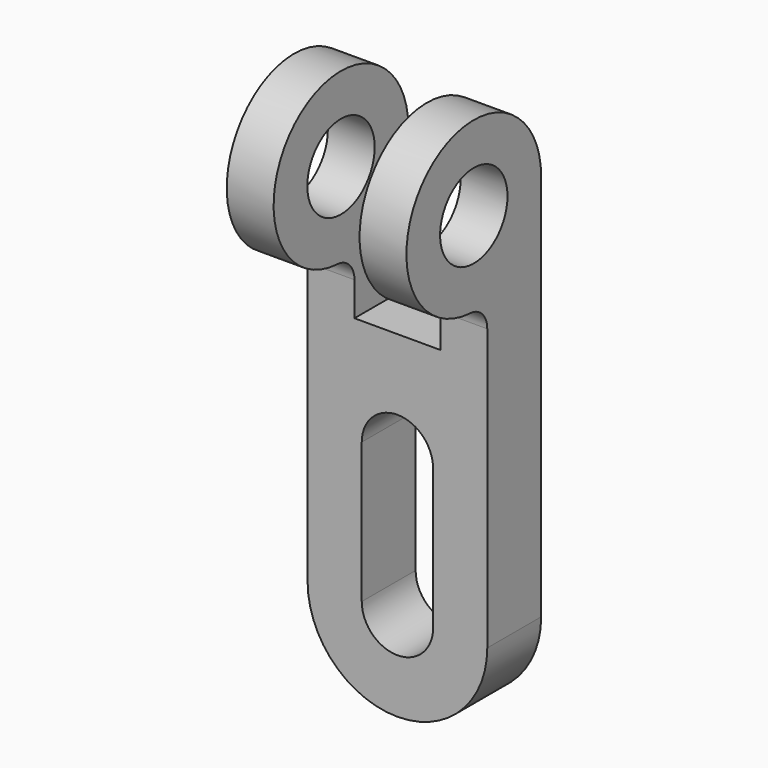
from build123d import *

# Parameters (mm, degrees)
F0_R     = 7.5
F1_DEPTH = 16
F3_W     = 15.3093371987
F3_H     = 50
F4_DEPTH = 55.501
F5_R     = 4
F6_DEPTH = 55.501


# Not quite as in the source:
# - a feature names something its author has since deleted; it is built from what else it names


with BuildPart() as f1:
    # F0 (on Right) → F1 (new body, symmetric)
    with BuildSketch(Plane.YZ):
        with BuildLine():
            Line((15, -85), (15, 0))
            ThreePointArc((15, 0), (-11.6189500386, 9.4868329805), (3, -14.6969384567))
            Line((3, -14.6969384567), (3, -85))
            Line((3, -85), (15, -85))
        make_face()
        Circle(F0_R, mode=Mode.SUBTRACT)
    extrude(amount=F1_DEPTH, both=True)

    # F3 (on offset) → F4 (cut, through all)
    with BuildSketch(Plane.XZ.offset(40.5)):
        with BuildLine():
            Line((6.3565325715, -68.9971852547), (6.3456283358, -44.3721764072))
            Line((6.3456283358, -44.3721764072), (6.3452962394, -43.6222039062))
            ThreePointArc((6.3452962394, -43.6222039062), (-0.1889815849, -37.6462766652), (-6.3565331947, -44))
            Line((-6.3565331947, -44), (-6.3565331947, -69))
            ThreePointArc((-6.3565331947, -69), (0, -75.3565331947), (6.3565331947, -69))
            ThreePointArc((6.3565331947, -69), (6.3565330389, -68.9985926273), (6.3565325715, -68.9971852547))
        make_face()
        Rectangle(F3_W, F3_H)
    extrude(amount=-F4_DEPTH, mode=Mode.SUBTRACT)

    # F5
    f5_edges = [f1.edges().sort_by_distance(p)[0] for p in [
        (-11.827334, 3, -14.696938),
        (11.827334, 3, -14.696938),
    ]]
    fillet(f5_edges, radius=F5_R)

    # F3 (on offset) → F6 (cut, through all)
    with BuildSketch(Plane.XZ.offset(40.5)):
        with BuildLine():
            ThreePointArc((2.313e-07, -85), (-11.3137084172, -80.3137085808), (-16, -69))
            Line((-16, -69), (-16, -85))
            Line((-16, -85), (2.313e-07, -85))
        make_face()
        with BuildLine():
            ThreePointArc((16, -69), (11.3137085808, -80.3137084172), (2.313e-07, -85))
            Line((2.313e-07, -85), (16, -85))
            Line((16, -85), (16, -69))
        make_face()
        with BuildLine():
            Line((6.3565325715, -68.9971852547), (6.3456283358, -44.3721764072))
            Line((6.3456283358, -44.3721764072), (6.3452962394, -43.6222039062))
            ThreePointArc((6.3452962394, -43.6222039062), (-0.1889815849, -37.6462766652), (-6.3565331947, -44))
            Line((-6.3565331947, -44), (-6.3565331947, -69))
            ThreePointArc((-6.3565331947, -69), (0, -75.3565331947), (6.3565331947, -69))
            ThreePointArc((6.3565331947, -69), (6.3565330389, -68.9985926273), (6.3565325715, -68.9971852547))
        make_face()
        Rectangle(F3_W, F3_H)
    extrude(amount=-F6_DEPTH, mode=Mode.SUBTRACT)


solid = f1.part
